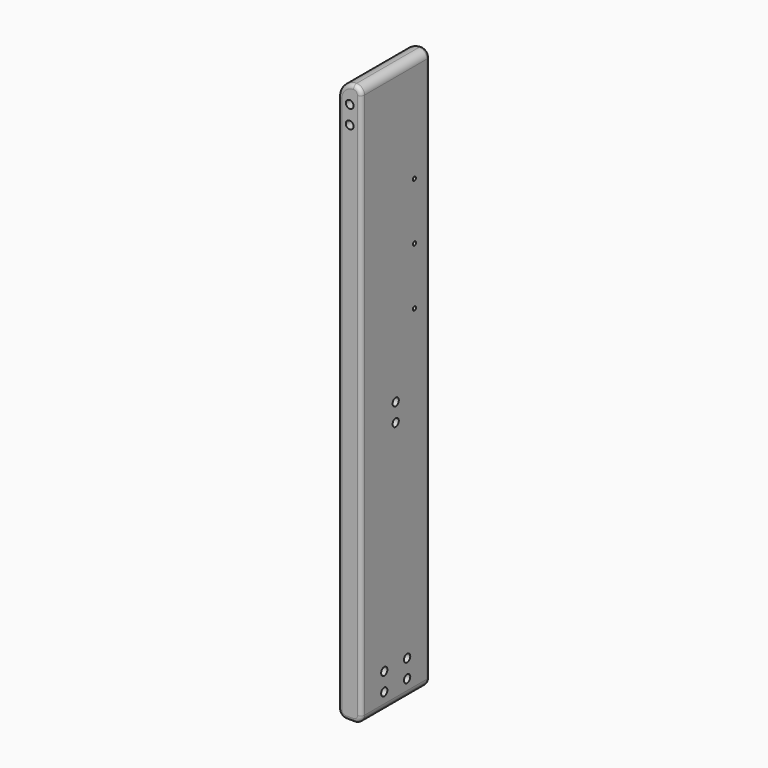
from build123d import *

# Parameters (mm, degrees)
F0_W        = 38.1
F0_H        = 914.4
F0_R        = 6.35
F1_DEPTH    = 139.7
F2_R        = 6.35
F3_DEPTH    = 38.1
F6_R        = 6.35
F7_DEPTH    = 38.1
F8_D        = 6.35
F4_R        = 12.7
F5_R        = 6.35
F9_T1_DEPTH = 139.7
F9_T4_ANGLE = 90
F9_T6_ANGLE = 90


# Not quite as in the source:
# - a fillet or chamfer that OpenCascade refuses, or shapes differently, is made with other operations: its cross-section is extruded or revolved along the edge and cut away or added


with BuildPart() as f1:
    # F0 (on Front) → F1 (new body)
    with BuildSketch(Plane.XZ):
        Rectangle(F0_W, F0_H)
        with Locations((0, 398.018)):
            Circle(F0_R, mode=Mode.SUBTRACT)
        with Locations((0, 427.482)):
            Circle(F0_R, mode=Mode.SUBTRACT)
    extrude(amount=-F1_DEPTH)

    # F2 (on face) → F3 (cut)
    with BuildSketch(Plane(origin=(-19.05, 0, 0), x_dir=(0, -1, 0), z_dir=(-1, 0, 0))):
        with Locations((-93.1418, -427.482)):
            Circle(F2_R)
        with Locations((-93.1418, -398.018)):
            Circle(F2_R)
        with Locations((-46.5836, -427.482)):
            Circle(F2_R)
        with Locations((-46.5836, -398.018)):
            Circle(F2_R)
    extrude(amount=-F3_DEPTH, mode=Mode.SUBTRACT)

    # F6 (on face) → F7 (cut)
    with BuildSketch(Plane(origin=(-19.05, 0, 0), x_dir=(0, -1, 0), z_dir=(-1, 0, 0))):
        with Locations((-69.85, -21.336)):
            Circle(F6_R)
        with Locations((-69.85, -50.8)):
            Circle(F6_R)
    extrude(amount=-F7_DEPTH, mode=Mode.SUBTRACT)

    # F8 (through all)
    with Locations(Plane(origin=(-19.05, 0, 0), x_dir=(0, -1, 0), z_dir=(-1, 0, 0))):
        with Locations((-107.95, 283.21), (-107.95, 190.246), (-107.95, 97.282)):
            Hole(F8_D / 2)

    # F4
    f4_edges = [f1.edges().sort_by_distance(p)[0] for p in [
        (19.05, 69.85, 457.2),
        (-19.05, 69.85, -457.2),
        (19.05, 69.85, -457.2),
    ]]
    fillet(f4_edges, radius=F4_R)

    # F5
    f5_edges = [f1.edges().sort_by_distance(p)[0] for p in [
        (-19.05, 0, 6.35),
        (19.05, 0, 0),
        (19.05, 139.7, 0),
    ]]
    fillet(f5_edges, radius=F5_R)

    # F9: fillet of radius 25.4 on 1 edges, made by hand

    # F9_s2 → F9_t1 (cut)
    with BuildSketch(Plane.XZ.offset(-139.7)):
        with BuildLine():
            ThreePointArc((6.35, 457.2), (-11.6105122421, 449.7605122421), (-19.05, 431.8))
            Line((-19.05, 431.8), (-19.05, 457.2))
            Line((-19.05, 457.2), (6.35, 457.2))
        make_face()
    extrude(amount=F9_T1_DEPTH, mode=Mode.SUBTRACT)

    # F9_s3 → F9_t4 (revolve, cut)
    with BuildSketch(Plane.YZ.offset(6.35)):
        with BuildLine():
            ThreePointArc((0, 450.85), (1.8598719395, 455.3401280605), (6.35, 457.2))
            Line((6.35, 457.2), (0, 457.2))
            Line((0, 457.2), (0, 450.85))
        make_face()
    revolve(axis=Axis((6.35, 0, 431.8), (0, -1, 0)), revolution_arc=F9_T4_ANGLE, mode=Mode.SUBTRACT)

    # F9_s5 → F9_t6 (revolve, cut)
    with BuildSketch(Plane.XY.offset(431.8)):
        with BuildLine():
            ThreePointArc((-12.7, 139.7), (-17.1901280605, 137.8401280605), (-19.05, 133.35))
            Line((-19.05, 133.35), (-19.05, 139.7))
            Line((-19.05, 139.7), (-12.7, 139.7))
        make_face()
    revolve(axis=Axis((6.35, 139.7, 431.8), (0, 1, 0)), revolution_arc=F9_T6_ANGLE, mode=Mode.SUBTRACT)


solid = f1.part
